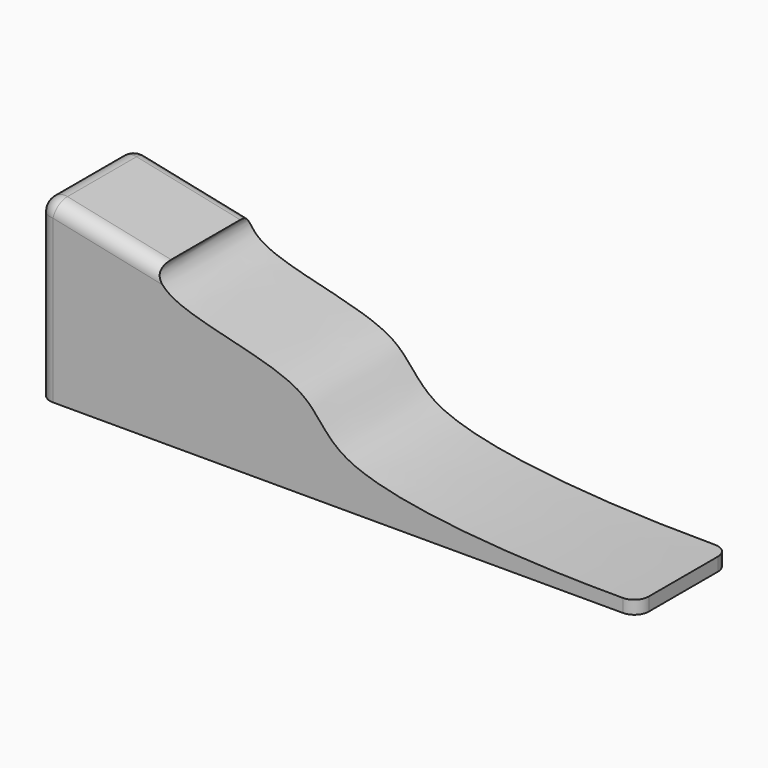
from build123d import *

# Parameters (mm, degrees)
F1_DEPTH = 40.64
F2_R     = 10.033
F3_DEPTH = 54.864
F5_DEPTH = 50.8
F10_R    = 5.08


# Not quite as in the source:
# - a feature of the source that left no trace in its solid (it failed there, or was rolled back) is left out


with BuildPart() as f1:
    # F0 (on Front) → F1 (new body)
    with BuildSketch(Plane.XZ):
        Polygon((0, 63.5), (0, 0), (211.2747204471, 0), (211.2747204471, 19.05), align=None)
    extrude(amount=-F1_DEPTH)

    # F2 (on face) → F3 (cut)
    with BuildSketch(Plane(origin=(0, 0, 0), x_dir=(0, -1, 0), z_dir=(-1, 0, 0))):
        with Locations((-20.9550000727, 31.3690006733)):
            Circle(F2_R)
    extrude(amount=-F3_DEPTH, mode=Mode.SUBTRACT)

    # F4 (on face) → F5 (cut)
    with BuildSketch(Plane.XZ):
        with BuildLine():
            Line((211.2747204471, 19.05), (42.7248373454, 54.5111393546))
            add(Edge.make_bspline(
                [(42.7248373454, 54.5111393546), (41.3835720379, 52.132302018), (45.7664482788, 42.0356948399), (97.7745530391, 36.833691871), (102.323893955, 6.8373724435), (182.6269030241, 4.3603729739), (211.2747204471, 4.6990001574)],
                knots=[0, 0, 0, 0, 0.0561852073, 0.1848977539, 0.2780173943, 0.468432753, 0.468432753, 0.468432753, 0.468432753], degree=3))
            Line((211.2747204471, 4.6990001574), (211.2747204471, 19.05))
        make_face()
    extrude(amount=-F5_DEPTH, mode=Mode.SUBTRACT)

    # F10
    f10_edges = [f1.edges().sort_by_distance(p)[0] for p in [
        (0, 0, 31.75),
        (21.362419, 0, 59.00557),
        (0, 20.32, 63.5),
        (21.362419, 40.64, 59.00557),
        (211.27472, 0, 2.3495),
        (0, 40.64, 31.75),
        (211.27472, 40.64, 2.3495),
    ]]
    fillet(f10_edges, radius=F10_R)


solid = f1.part
